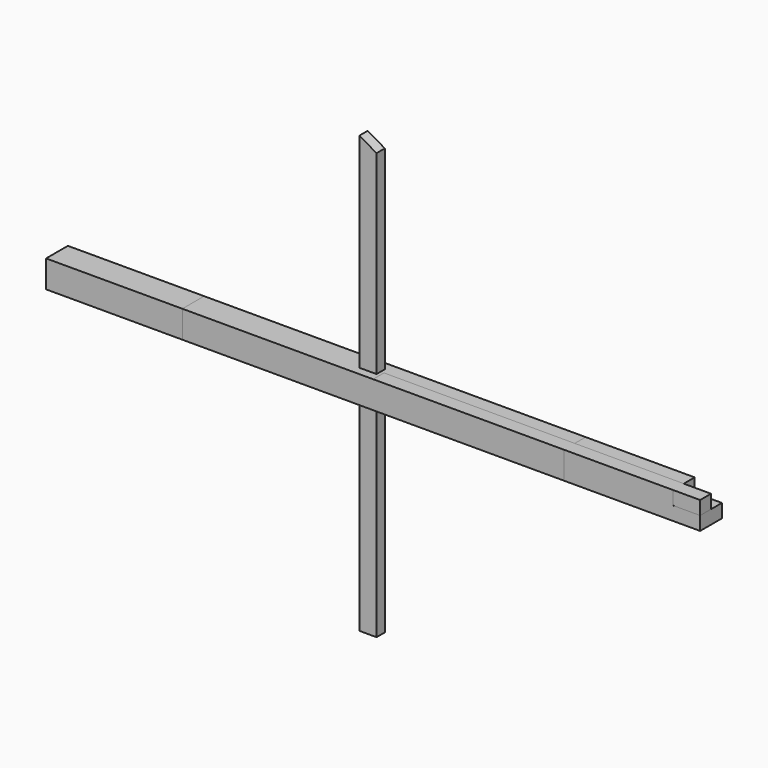
from build123d import *

# Parameters (mm, degrees)
F1_DEPTH = 50
F2_W     = 1400
F2_H     = 100
F3_DEPTH = 50
F4_W     = 63
F4_H     = 1600
F5_DEPTH = 19
F6_SIZE2 = 36.373057
F6_SIZE  = 62.99999
F7_W     = 50
F7_H     = 50
F8_DEPTH = 1200


# Not quite as in the source:
# - a fillet or chamfer is up to 0.001 mm smaller than in the source, because OpenCascade refuses the exact size


with BuildPart() as f1:
    # F0 (on Front) → F1 (new body, symmetric)
    with BuildSketch(Plane.XZ):
        Polygon((1100, 0), (1100, 50), (-1200, 50), (-1200, -50), (1200, -50), (1200, 0), align=None)
    extrude(amount=F1_DEPTH, both=True)


with BuildPart() as f3:
    # F2 (on Front) → F3 (new body, symmetric)
    with BuildSketch(Plane.XZ):
        Rectangle(F2_W, F2_H)
    extrude(amount=F3_DEPTH, both=True)


with BuildPart() as f5:
    # F4 (on Front) → F5 (new body, symmetric)
    with BuildSketch(Plane.XZ):
        with Locations((-43.6704657625, 0)):
            Rectangle(F4_W, F4_H)
    extrude(amount=F5_DEPTH, both=True)

    # F6 (size 63 and 36.3730669589 in the source; OpenCascade refuses exactly that, so slightly less here)
    f6_edges = [f5.edges().sort_by_distance(p)[0] for p in [
        (-12.170466, 0, 800),
    ]]
    f6_side = f5.faces().sort_by_distance((-43.670466, 0, 800))[0]
    chamfer(f6_edges, length=F6_SIZE, length2=F6_SIZE2, reference=f6_side)


with BuildPart() as f8:
    # F7 (on Right) → F8 (new body)
    with BuildSketch(Plane.YZ):
        with Locations((-24.9985475093, 25)):
            Rectangle(F7_W, F7_H)
    extrude(amount=F8_DEPTH)


solid = Compound([f1.part, f3.part, f5.part, f8.part])
